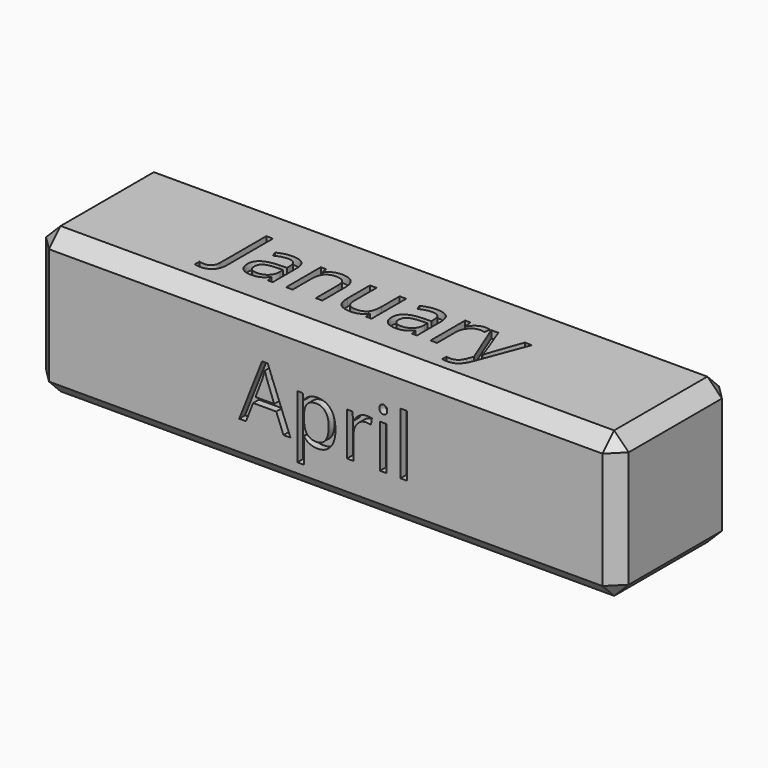
from build123d import *

# Parameters (mm, degrees)
F0_W          = 101.6
F0_H          = 25.4
F1_DEPTH      = 12.7
F1_DEPTH_BACK = 12.7
F2_SIZE       = 2.54
F3_TEXT_SIZE  = 14.1111111111
F4_DEPTH      = 1.27
F5_TEXT_SIZE  = 14.1111111111
F6_DEPTH      = 1.27
F7_TEXT_SIZE  = 14.1111111111
F8_DEPTH      = 1.27
F9_TEXT_SIZE  = 14.1111111111
F10_DEPTH     = 1.27


# Not quite as in the source:
# - Text() gives the source's letters only with a copy of the font that has no kerning and outlines rounded to 1/6400 em; it was checked with that copy


with BuildPart() as f1:
    # F0 (on Top) → F1 (new body, two sides)
    with BuildSketch(Plane.XY) as f1_sk:
        Rectangle(F0_W, F0_H)
    extrude(amount=F1_DEPTH)
    extrude(f1_sk.sketch, amount=-F1_DEPTH_BACK)

    # F2
    f2_edges = [f1.edges().sort_by_distance(p)[0] for p in [
        (50.8, 0, 12.7),
        (0, 12.7, 12.7),
        (-50.8, 0, 12.7),
        (0, -12.7, 12.7),
        (-50.8, 12.7, 0),
        (0, 12.7, -12.7),
        (50.8, 12.7, 0),
        (-50.8, -12.7, 0),
        (-50.8, 0, -12.7),
        (50.8, 0, -12.7),
        (0, -12.7, -12.7),
        (50.8, -12.7, 0),
    ]]
    chamfer(f2_edges, length=F2_SIZE)

    # F3 (on face) → F4 (cut)
    with BuildSketch(Plane.XY.offset(12.7)):
        with Locations((-25.8299479167, -5.08)):
            Text('January', F3_TEXT_SIZE, font='Open Sans', text_align=(TextAlign.LEFT, TextAlign.BOTTOM))
    extrude(amount=-F4_DEPTH, mode=Mode.SUBTRACT)

    # F5 (on face) → F6 (cut)
    with BuildSketch(Plane(origin=(0, 12.7, 0), x_dir=(-1, 0, 0), z_dir=(0, 1, 0))):
        with Locations(Location((29.9453211806, 5.08), (0, 0, -180))):
            Text('February', F5_TEXT_SIZE, font='Open Sans', text_align=(TextAlign.LEFT, TextAlign.BOTTOM))
    extrude(amount=-F6_DEPTH, mode=Mode.SUBTRACT)

    # F7 (on face) → F8 (cut)
    with BuildSketch(Plane(origin=(0, 0, -12.7), x_dir=(1, 0, 0), z_dir=(0, 0, -1))):
        with Locations((-20.7532552083, -5.08)):
            Text('March', F7_TEXT_SIZE, font='Open Sans', text_align=(TextAlign.LEFT, TextAlign.BOTTOM))
    extrude(amount=-F8_DEPTH, mode=Mode.SUBTRACT)

    # F9 (on face) → F10 (cut)
    with BuildSketch(Plane.XZ.offset(12.7)):
        with Locations((-15.0900694444, -5.08)):
            Text('April', F9_TEXT_SIZE, font='Open Sans', text_align=(TextAlign.LEFT, TextAlign.BOTTOM))
    extrude(amount=-F10_DEPTH, mode=Mode.SUBTRACT)


solid = f1.part
